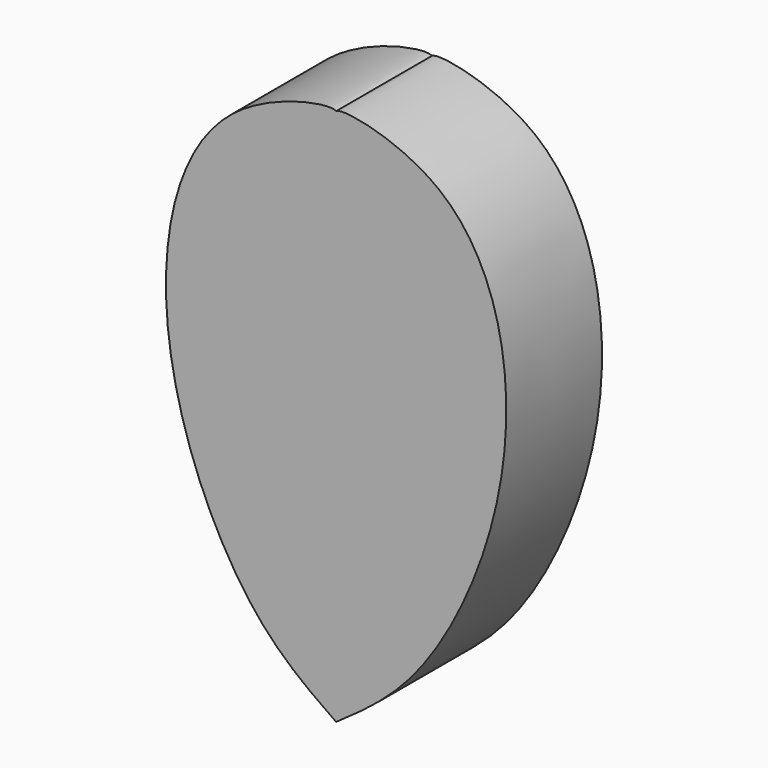
from build123d import *

# Parameters (mm, degrees)
F1_DEPTH = 25.4


with BuildPart() as f1:
    # F0 (on Front) → F1 (new body)
    with BuildSketch(Plane.XZ):
        with BuildLine():
            add(Edge.make_bspline(
                [(0, -39.4752658904), (-5.9743297577, -35.3221398514), (-20.5901420925, -25.1617645997), (-41.4083426371, 21.2933695148), (-30.9811462178, 70.3817835785), (-1.4680619477, 75.739568974), (0, 74.6092498302)],
                knots=[0, 0, 0, 0, 0.1981423854, 0.4847433144, 0.7633618557, 0.9597199549, 0.9597199549, 0.9597199549, 0.9597199549], degree=3))
            Line((0, -39.4752658904), (0, 73.6320614815))
            add(Edge.make_bspline(
                [(0, 74.6092498302), (-0.3011518332, 74.3773810847), (-0.1506598826, 74.0047417367), (0, 73.6320614815)],
                knots=[0.9597199549, 0.9597199549, 0.9597199549, 0.9597199549, 1, 1, 1, 1], degree=3))
        make_face()
        with BuildLine():
            Line((0, 73.6320614815), (0, -39.4752658904))
            add(Edge.make_bspline(
                [(0, -39.4752658904), (5.9743297577, -35.3221398514), (20.5901420925, -25.1617645997), (41.4083426371, 21.2933695148), (30.9811462178, 70.3817835785), (1.4680619477, 75.739568974), (0, 74.6092498302)],
                knots=[0, 0, 0, 0, 0.1981423854, 0.4847433144, 0.7633618557, 0.9597199549, 0.9597199549, 0.9597199549, 0.9597199549], degree=3))
            add(Edge.make_bspline(
                [(0, 74.6092498302), (0.3011518332, 74.3773810847), (0.1506598826, 74.0047417367), (0, 73.6320614815)],
                knots=[0.9597199549, 0.9597199549, 0.9597199549, 0.9597199549, 1, 1, 1, 1], degree=3))
        make_face()
        with BuildLine():
            add(Edge.make_bspline(
                [(0, 74.6092498302), (0.3011518332, 74.3773810847), (0.1506598826, 74.0047417367), (0, 73.6320614815)],
                knots=[0.9597199549, 0.9597199549, 0.9597199549, 0.9597199549, 1, 1, 1, 1], degree=3))
            Line((0, 74.6092498302), (0, 73.6320614815))
        make_face()
        with BuildLine():
            Line((0, 73.6320614815), (0, 74.6092498302))
            add(Edge.make_bspline(
                [(0, 74.6092498302), (-0.3011518332, 74.3773810847), (-0.1506598826, 74.0047417367), (0, 73.6320614815)],
                knots=[0.9597199549, 0.9597199549, 0.9597199549, 0.9597199549, 1, 1, 1, 1], degree=3))
        make_face()
    extrude(amount=F1_DEPTH)


solid = f1.part
